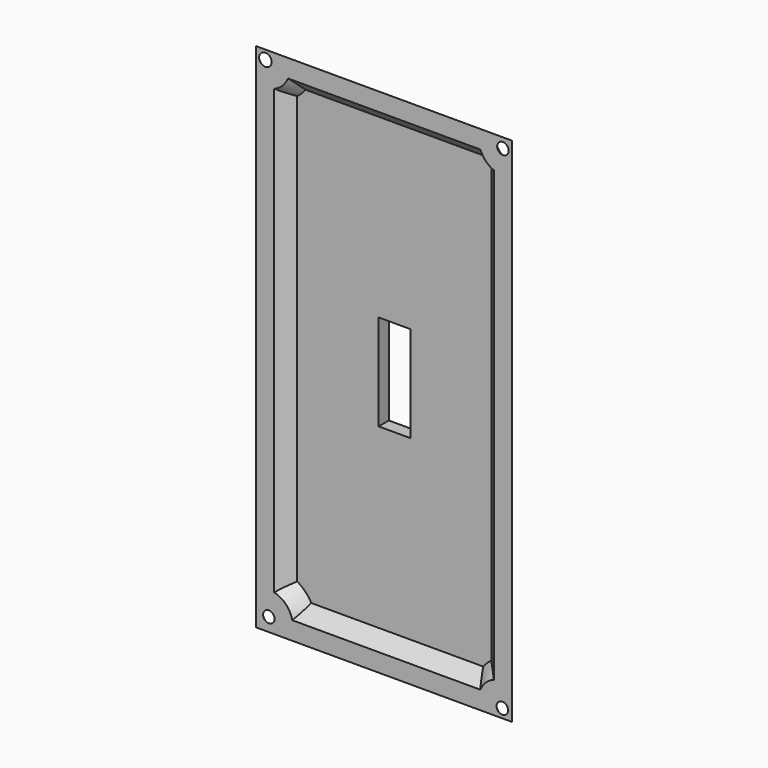
from build123d import *

# Parameters (mm, degrees)
F0_W        = 50.8
F0_H        = 101.6
F0_R        = 1.143
F0_R_2      = 1.2394927364
F1_DEPTH    = 5.08
F2_T1_DEPTH = 127.7282991577
F2_T3_DEPTH = 76.9282991577
F3_T        = -2.54
F4_W        = 6.35
F4_H        = 19.05
F5_DEPTH    = 25.4


# Not quite as in the source:
# - a fillet or chamfer that OpenCascade refuses, or shapes differently, is made with other operations: its cross-section is extruded or revolved along the edge and cut away or added


with BuildPart() as f1:
    # F0 (on Front) → F1 (new body)
    with BuildSketch(Plane.XZ):
        with Locations((-0.076776122, -0.0760140894)):
            Rectangle(F0_W, F0_H)
        with Locations((-22.936776122, -48.2090140894)):
            Circle(F0_R, mode=Mode.SUBTRACT)
        with Locations((23.418223878, -49.0980140894)):
            Circle(F0_R, mode=Mode.SUBTRACT)
        with Locations((-23.6282116387, 48.9378400757)):
            Circle(F0_R_2, mode=Mode.SUBTRACT)
        with Locations((23.5306444928, 48.7492585503)):
            Circle(F0_R, mode=Mode.SUBTRACT)
    extrude(amount=F1_DEPTH)

    # F2: chamfer of 5.08 on 8 edges, made by hand

    # F2_s2 → F2_t1 (cut)
    with BuildSketch(Plane.XY.offset(-63.9401636683)):
        Polygon((25.323223878, -5.08), (20.243223878, 0), (25.323223878, 0), align=None)
        Polygon((-25.476776122, -5.08), (-20.396776122, 0), (-25.476776122, 0), align=None)
    extrude(amount=F2_T1_DEPTH, mode=Mode.SUBTRACT)

    # F2_s4 → F2_t3 (cut)
    with BuildSketch(Plane.YZ.offset(-38.5409257009)):
        Polygon((-5.08, 50.7239859106), (0, 45.6439859106), (0, 50.7239859106), align=None)
        Polygon((-5.08, -50.8760140894), (0, -45.7960140894), (0, -50.8760140894), align=None)
    extrude(amount=F2_T3_DEPTH, mode=Mode.SUBTRACT)

    # F2_s5 → F2_t6 (revolve, cut)
    with BuildSketch(Plane.XY.offset(48.9378400757)):
        Polygon((-22.3887189023, -5.08), (-17.3087189023, 0), (-22.3887189023, 0), align=None)
    revolve(axis=Axis((-23.6282116387, 0, 48.9378400757), (0, -1, 0)), mode=Mode.SUBTRACT)

    # F2_s7 → F2_t8 (revolve, cut)
    with BuildSketch(Plane.XY.offset(48.7492585503)):
        Polygon((24.6736444928, -5.08), (29.7536444928, 0), (24.6736444928, 0), align=None)
    revolve(axis=Axis((23.5306444928, 0, 48.7492585503), (0, -1, 0)), mode=Mode.SUBTRACT)

    # F2_s9 → F2_t10 (revolve, cut)
    with BuildSketch(Plane.XY.offset(-48.2090140894)):
        Polygon((-21.793776122, -5.08), (-16.713776122, 0), (-21.793776122, 0), align=None)
    revolve(axis=Axis((-22.936776122, 0, -48.2090140894), (0, -1, 0)), mode=Mode.SUBTRACT)

    # F2_s11 → F2_t12 (revolve, cut)
    with BuildSketch(Plane.XY.offset(-49.0980140894)):
        Polygon((24.561223878, -5.08), (29.641223878, 0), (24.561223878, 0), align=None)
    revolve(axis=Axis((23.418223878, 0, -49.0980140894), (0, -1, 0)), mode=Mode.SUBTRACT)

    # F3
    f3_openings = [f1.faces().sort_by_distance(p)[0] for p in [
        (-0.074021, -5.08, -0.083441),
    ]]
    offset(amount=F3_T, openings=f3_openings)

    # F4 (on face) → F5 (cut)
    with BuildSketch(Plane(origin=(0, 0, 0), x_dir=(-1, 0, 0), z_dir=(0, 1, 0))):
        Rectangle(F4_W, F4_H)
    extrude(amount=-F5_DEPTH, mode=Mode.SUBTRACT)


solid = f1.part
